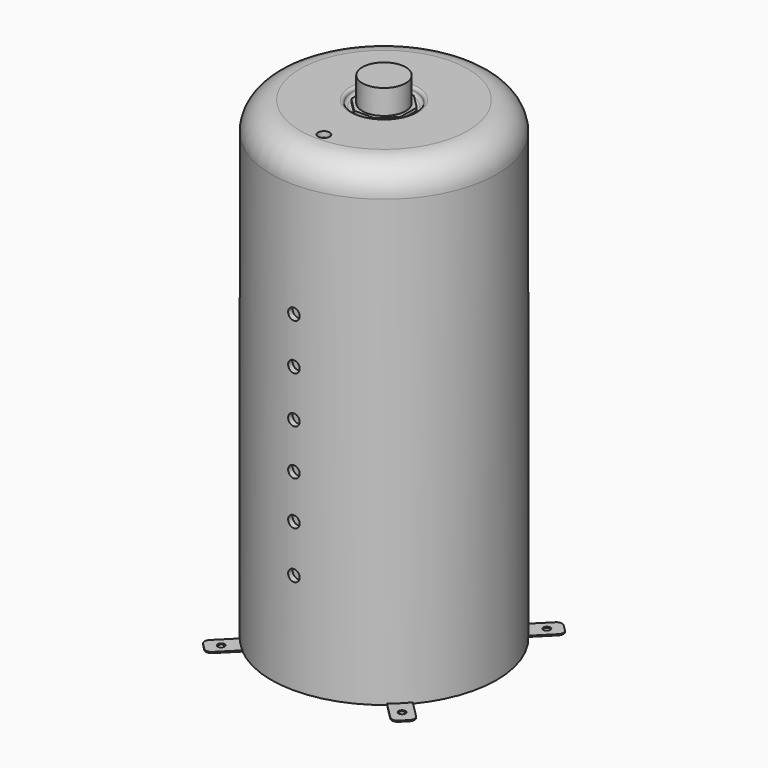
from build123d import *

# Parameters (mm, degrees)
F3_R      = 54
F4_DEPTH  = 10
F5_R      = 4.99999
F7_DEPTH  = 5
F8_R      = 37.5
F9_DEPTH  = 37.5
F11_R     = 10
F12_DEPTH = 10
F13_R     = 10
F14_DEPTH = 10
F15_R     = 6
F16_DEPTH = 2


# Not quite as in the source:
# - a fillet or chamfer is up to 0.001 mm smaller than in the source, because OpenCascade refuses the exact size


with BuildPart() as f2:
    # F1 (on Front) → F2 (revolve)
    with BuildSketch(Plane.XZ):
        with BuildLine():
            Line((0, 820), (0, 0))
            Line((0, 0), (195, 0))
            Line((195, 0), (195, 770))
            ThreePointArc((195, 770), (180.3553390593, 805.3553390593), (145, 820))
            Line((145, 820), (0, 820))
        make_face()
    revolve(axis=Axis((0, 0, 410), (0, 0, -1)))

    # F3 (on face) → F4 (cut)
    with BuildSketch(Plane.XY.offset(820)):
        Circle(F3_R)
    extrude(amount=-F4_DEPTH, mode=Mode.SUBTRACT)

    # F5 (radius 5 in the source; OpenCascade refuses exactly that, so slightly less here)
    f5_edges = [f2.edges().sort_by_distance(p)[0] for p in [
        (-54, 0, 820),
        (-54, 0, 810),
    ]]
    fillet(f5_edges, radius=F5_R)

    # F6 (on face) → F7 (join)
    with BuildSketch(Plane.XY.offset(810)):
        Polygon((-17.6040764009, -42.5), (17.6040764009, -42.5), (42.5, -17.6040764009), (42.5, 17.6040764009), (17.6040764009, 42.5), (-17.6040764009, 42.5), (-42.5, 17.6040764009), (-42.5, -17.6040764009), align=None)
    extrude(amount=F7_DEPTH)

    # F8 (on face) → F9 (join, symmetric)
    with BuildSketch(Plane.XY.offset(820)):
        Circle(F8_R)
    extrude(amount=F9_DEPTH, both=True)

    # F11 (on offset) → F12 (cut)
    with BuildSketch(Plane.XZ.offset(195)):
        with Locations((0, 175)):
            Circle(F11_R)
        with Locations((0, 257)):
            Circle(F11_R)
        with Locations((0, 333)):
            Circle(F11_R)
        with Locations((0, 412)):
            Circle(F11_R)
        with Locations((0, 493)):
            Circle(F11_R)
        with Locations((0, 573)):
            Circle(F11_R)
    extrude(amount=-F12_DEPTH, mode=Mode.SUBTRACT)

    # F13 (on face) → F14 (cut)
    with BuildSketch(Plane.XY.offset(820)):
        with Locations((0, -130)):
            Circle(F13_R)
    extrude(amount=-F14_DEPTH, mode=Mode.SUBTRACT)

    # F15 (on face) → F16 (join)
    with BuildSketch(Plane(origin=(0, 0, 0), x_dir=(1, 0, 0), z_dir=(0, 0, -1))):
        with BuildLine():
            ThreePointArc((-153.7957249081, 178.5444622496), (-160.8667927199, 181.4733944377), (-167.9378605318, 178.5444622496))
            Line((-167.9378605318, 178.5444622496), (-178.5444622496, 167.9378605318))
            ThreePointArc((-178.5444622496, 167.9378605318), (-181.4733944377, 160.8667927199), (-178.5444622496, 153.7957249081))
            Line((-178.5444622496, 153.7957249081), (-146.1599508606, 121.411213519))
            Line((-146.1599508606, 121.411213519), (-121.411213519, 146.1599508606))
            Line((-121.411213519, 146.1599508606), (-153.7957249081, 178.5444622496))
        make_face()
        with Locations((-156.4564352241, 156.4564352241)):
            Circle(F15_R, mode=Mode.SUBTRACT)
        with BuildLine():
            Line((-153.7957249081, -178.5444622496), (-121.411213519, -146.1599508606))
            Line((-121.411213519, -146.1599508606), (-146.1599508606, -121.411213519))
            Line((-146.1599508606, -121.411213519), (-178.5444622496, -153.7957249081))
            ThreePointArc((-178.5444622496, -153.7957249081), (-181.4733944377, -160.8667927199), (-178.5444622496, -167.9378605318))
            Line((-178.5444622496, -167.9378605318), (-167.9378605318, -178.5444622496))
            ThreePointArc((-167.9378605318, -178.5444622496), (-160.8667927199, -181.4733944377), (-153.7957249081, -178.5444622496))
        make_face()
        with Locations((-156.4564352241, -156.4564352241)):
            Circle(F15_R, mode=Mode.SUBTRACT)
        with BuildLine():
            Line((178.5444622496, -153.7957249081), (146.1599508606, -121.411213519))
            Line((146.1599508606, -121.411213519), (121.411213519, -146.1599508606))
            Line((121.411213519, -146.1599508606), (153.7957249081, -178.5444622496))
            ThreePointArc((153.7957249081, -178.5444622496), (160.8667927199, -181.4733944377), (167.9378605318, -178.5444622496))
            Line((167.9378605318, -178.5444622496), (178.5444622496, -167.9378605318))
            ThreePointArc((178.5444622496, -167.9378605318), (181.4733944377, -160.8667927199), (178.5444622496, -153.7957249081))
        make_face()
        with Locations((156.4564352241, -156.4564352241)):
            Circle(F15_R, mode=Mode.SUBTRACT)
        with BuildLine():
            Line((153.7957249081, 178.5444622496), (121.411213519, 146.1599508606))
            Line((121.411213519, 146.1599508606), (146.1599508606, 121.411213519))
            Line((146.1599508606, 121.411213519), (178.5444622496, 153.7957249081))
            ThreePointArc((178.5444622496, 153.7957249081), (181.4733944377, 160.8667927199), (178.5444622496, 167.9378605318))
            Line((178.5444622496, 167.9378605318), (167.9378605318, 178.5444622496))
            ThreePointArc((167.9378605318, 178.5444622496), (160.8667927199, 181.4733944377), (153.7957249081, 178.5444622496))
        make_face()
        with Locations((156.4564352241, 156.4564352241)):
            Circle(F15_R, mode=Mode.SUBTRACT)
    extrude(amount=-F16_DEPTH)


solid = f2.part
